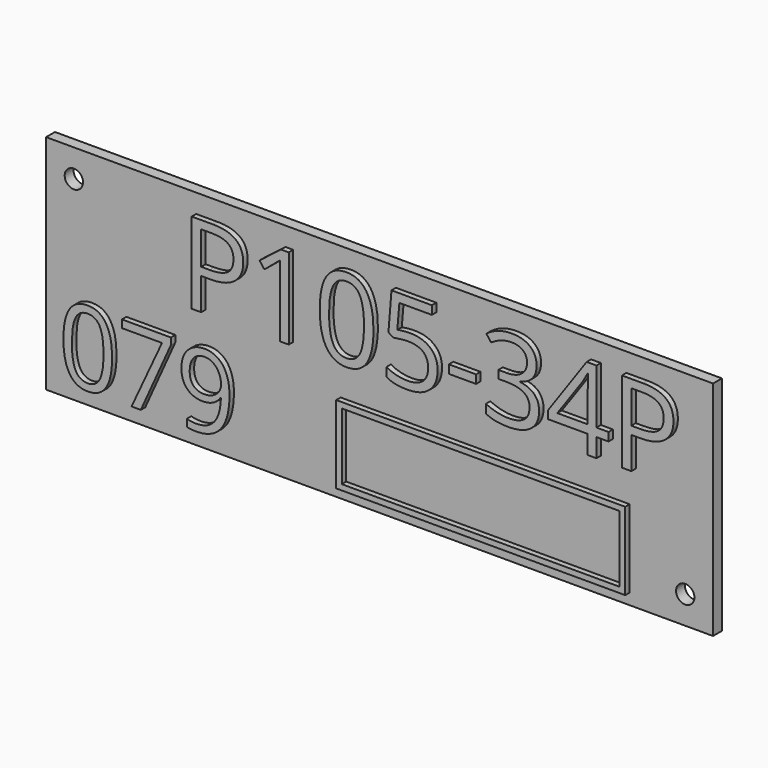
from build123d import *

# Parameters (mm, degrees)
F0_W         = 120
F0_H         = 40
F1_DEPTH     = 2
F3_D         = 3.3
F4_TEXT_SIZE = 20.4639926102
F5_DEPTH     = 1
F6_TEXT_SIZE = 18.5356140827
F7_DEPTH     = 1
F8_W         = 52
F8_H         = 14
F8_W_2       = 49.99999962
F8_H_2       = 11.99999962
F9_DEPTH     = 1


# Not quite as in the source:
# - Text() gives the source's letters only with a copy of the font that has no kerning and outlines rounded to 1/6400 em; it was checked with that copy


with BuildPart() as f1:
    # F0 (on Front) → F1 (new body)
    with BuildSketch(Plane.XZ):
        Rectangle(F0_W, F0_H)
    extrude(amount=F1_DEPTH)

    # F3 (through all)
    with Locations(Plane.XZ.offset(2)):
        with Locations((-55, 15), (55, -15)):
            Hole(F3_D / 2)

    # F4 (on face) → F5 (join)
    with BuildSketch(Plane.XZ.offset(2)):
        with Locations((-35, 2)):
            Text('P105-34P', F4_TEXT_SIZE, font='Open Sans', text_align=(TextAlign.LEFT, TextAlign.BOTTOM))
    extrude(amount=F5_DEPTH)

    # F6 (on face) → F7 (join)
    with BuildSketch(Plane.XZ.offset(2)):
        with Locations((-57, -17)):
            Text('079', F6_TEXT_SIZE, font='Open Sans', text_align=(TextAlign.LEFT, TextAlign.BOTTOM))
    extrude(amount=F7_DEPTH)

    # F8 (on face) → F9 (join)
    with BuildSketch(Plane.XZ.offset(2)):
        with Locations((19, -11)):
            Rectangle(F8_W, F8_H)
        with Locations((19, -11)):
            Rectangle(F8_W_2, F8_H_2, mode=Mode.SUBTRACT)
    extrude(amount=F9_DEPTH)


solid = f1.part
